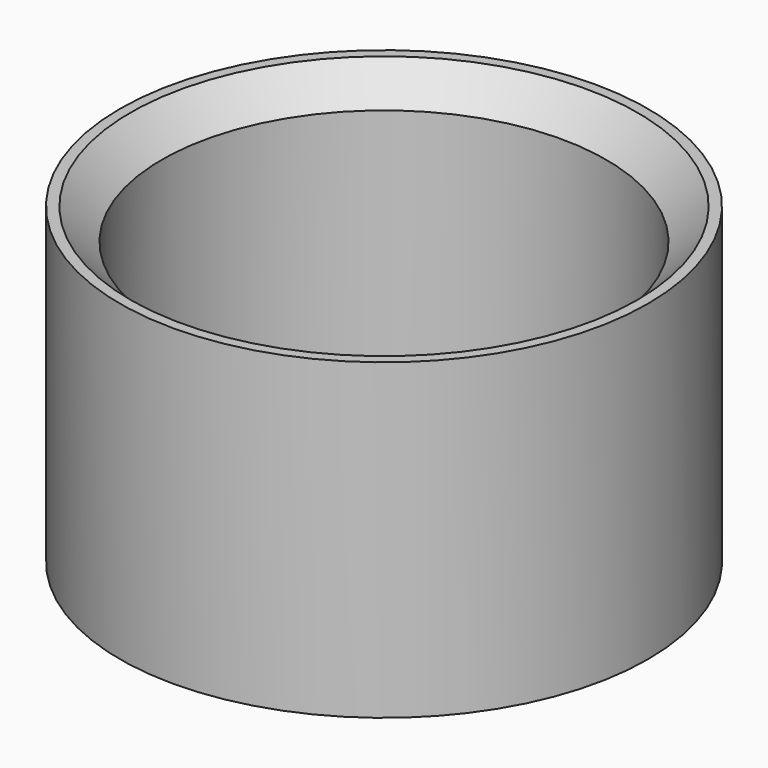
from build123d import *

# Parameters (mm, degrees)
F0_R     = 12.65
F1_DEPTH = 15
F2_T     = -2
F3_SIZE  = 1.5


with BuildPart() as f1:
    # F0 (on Top) → F1 (new body)
    with BuildSketch(Plane.XY):
        Circle(F0_R)
    extrude(amount=F1_DEPTH)

    # F2
    f2_openings = [f1.faces().sort_by_distance(p)[0] for p in [
        (0, 0, 15),
    ]]
    offset(amount=F2_T, openings=f2_openings)

    # F3
    f3_edges = [f1.edges().sort_by_distance(p)[0] for p in [
        (-10.65, 0, 15),
    ]]
    chamfer(f3_edges, length=F3_SIZE)


solid = f1.part
